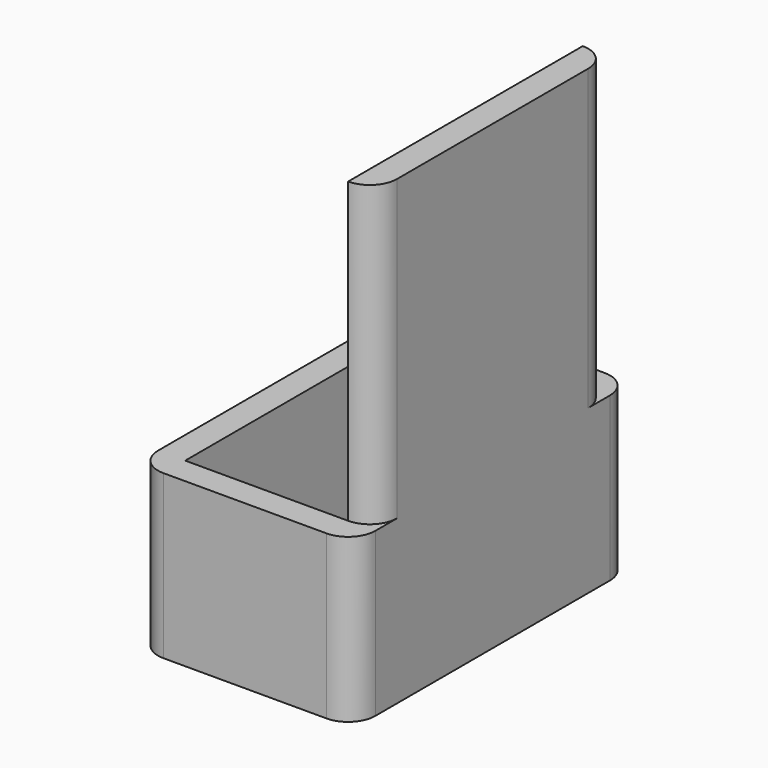
from build123d import *

# Parameters (mm, degrees)
F0_W     = 5
F0_H     = 54
F1_DEPTH = 85
F0_W_2   = 30
F2_DEPTH = 5
F3_DEPTH = 30
F4_R     = 4.99999


# Not quite as in the source:
# - a fillet or chamfer is up to 0.001 mm smaller than in the source, because OpenCascade refuses the exact size


with BuildPart() as f1:
    # F0 (on Top) → F1 (new body)
    with BuildSketch(Plane.XY):
        with Locations((17.5, 0)):
            Rectangle(F0_W, F0_H)
    extrude(amount=F1_DEPTH)

    # F0 (on Top) → F2 (join)
    with BuildSketch(Plane.XY):
        Rectangle(F0_W_2, F0_H)
    extrude(amount=F2_DEPTH)

    # F0 (on Top) → F3 (join)
    with BuildSketch(Plane.XY):
        Polygon((20, -27), (15, -27), (-15, -27), (-15, 27), (15, 27), (20, 27), (20, 32), (-20, 32), (-20, -31.9579449729), (-20, -32), (20, -32), align=None)
    extrude(amount=F3_DEPTH)

    # F4 (radius 5 in the source; OpenCascade refuses exactly that, so slightly less here)
    f4_edges = [f1.edges().sort_by_distance(p)[0] for p in [
        (-20, -32, 15),
        (20, -32, 15),
        (20, 32, 15),
        (-20, 32, 15),
        (20, 27, 57.5),
        (20, -27, 57.5),
    ]]
    fillet(f4_edges, radius=F4_R)


solid = f1.part
